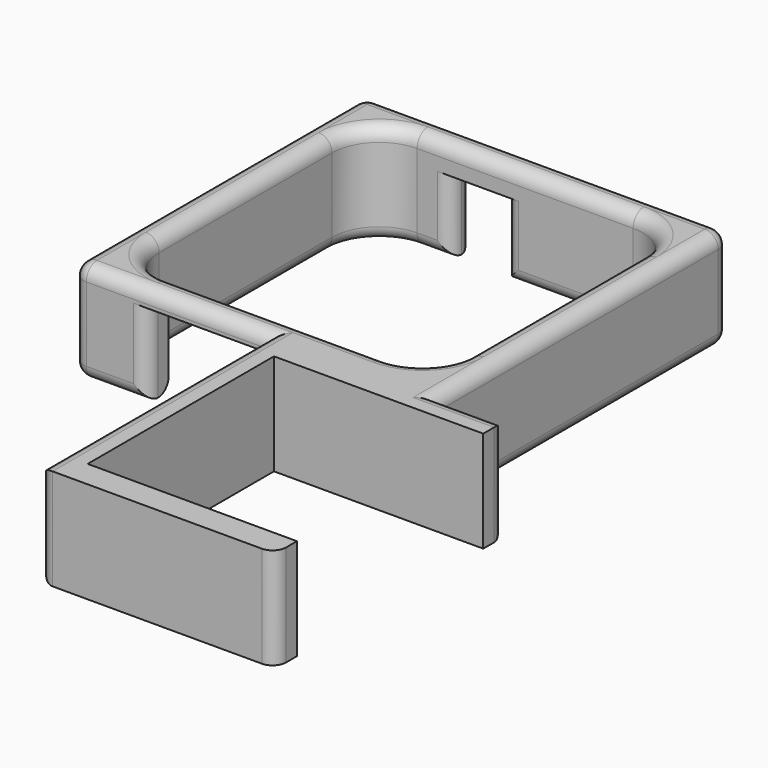
from build123d import *

# Parameters (mm, degrees)
F1_DEPTH = 7.5
F2_W     = 18
F2_H     = 4
F2_W_2   = 8
F3_DEPTH = 7.5
F4_DEPTH = 5
F5_DEPTH = 25
F6_DEPTH = 3.5
F7_DEPTH = 25
F8_R     = 7
F9_R     = 1.99999


# Not quite as in the source:
# - a fillet or chamfer is up to 0.001 mm smaller than in the source, because OpenCascade refuses the exact size


with BuildPart() as f1:
    # F0 (on Top) → F1 (new body, symmetric)
    with BuildSketch(Plane.XY):
        Polygon((29.4704200836, 10.5355388032), (29.4704200836, 14.5355388032), (-5.5295799164, 14.5355388032), (-5.5295799164, -27.9644611968), (29.4704200836, -27.9644611968), (29.4704200836, -23.9644611968), (27.4704200836, -23.9644611968), (-1.5295799164, -23.9644611968), (-1.5295799164, 10.5355388032), (27.4704200836, 10.5355388032), align=None)
    extrude(amount=F1_DEPTH, both=True)

    # F2 (on Top) → F3 (join, symmetric)
    with BuildSketch(Plane.XY):
        Polygon((-30.5295799164, 18.5355388032), (-30.5295799164, 64.5355388032), (-18.5295799164, 64.5355388032), (-18.5295799164, 68.5355388032), (-34.5295799164, 68.5355388032), (-34.5295799164, 14.5355388032), (-23.5295799164, 14.5355388032), (-23.5295799164, 18.5355388032), align=None)
        Polygon((-10.5295799164, 68.5355388032), (-10.5295799164, 64.5355388032), (15.4704200836, 64.5355388032), (15.4704200836, 18.5355388032), (-5.5295799164, 18.5355388032), (-5.5295799164, 14.5355388032), (19.4704200836, 14.5355388032), (19.4704200836, 68.5355388032), align=None)
        with Locations((-14.5295799164, 16.5355388032)):
            Rectangle(F2_W, F2_H)
        with Locations((-14.5295799164, 66.5355388032)):
            Rectangle(F2_W_2, F2_H)
    extrude(amount=F3_DEPTH, both=True)

    # F2 (on Top) → F4 (cut, symmetric)
    with BuildSketch(Plane.XY):
        with Locations((-14.5295799164, 16.5355388032)):
            Rectangle(F2_W, F2_H)
    extrude(amount=F4_DEPTH, both=True, mode=Mode.SUBTRACT)

    # F2 (on Top) → F5 (cut)
    with BuildSketch(Plane.XY):
        with Locations((-14.5295799164, 16.5355388032)):
            Rectangle(F2_W, F2_H)
    extrude(amount=-F5_DEPTH, mode=Mode.SUBTRACT)

    # F2 (on Top) → F6 (cut, symmetric)
    with BuildSketch(Plane.XY):
        with Locations((-14.5295799164, 66.5355388032)):
            Rectangle(F2_W_2, F2_H)
    extrude(amount=F6_DEPTH, both=True, mode=Mode.SUBTRACT)

    # F2 (on Top) → F7 (cut)
    with BuildSketch(Plane.XY):
        with Locations((-14.5295799164, 66.5355388032)):
            Rectangle(F2_W_2, F2_H)
    extrude(amount=-F7_DEPTH, mode=Mode.SUBTRACT)

    # F8
    f8_edges = [f1.edges().sort_by_distance(p)[0] for p in [
        (-30.52958, 64.535539, 0),
        (15.47042, 64.535539, 0),
        (-30.52958, 18.535539, 0),
        (15.47042, 18.535539, 0),
    ]]
    fillet(f8_edges, radius=F8_R)

    # F9 (radius 2 in the source; OpenCascade refuses exactly that, so slightly less here)
    f9_edges = [f1.edges().sort_by_distance(p)[0] for p in [
        (19.47042, 41.535539, 7.5),
        (19.47042, 41.535539, -7.5),
        (24.47042, 14.535539, 7.5),
        (24.47042, 14.535539, -7.5),
        (19.47042, 68.535539, 0),
        (4.47042, 68.535539, -7.5),
        (-7.52958, 68.535539, 7.5),
        (-14.52958, 68.535539, 3.5),
        (-18.52958, 68.535539, -2),
        (-10.52958, 68.535539, -2),
        (-10.52958, 64.535539, -2),
        (-18.52958, 64.535539, -2),
        (-34.52958, 68.535539, 0),
        (-26.52958, 68.535539, -7.5),
        (-30.52958, 41.535539, -7.5),
        (15.47042, 41.535539, -7.5),
        (-34.52958, 41.535539, -7.5),
        (-29.02958, 14.535539, -7.5),
        (-34.52958, 41.535539, 7.5),
        (-20.02958, 14.535539, 7.5),
        (-30.52958, 41.535539, 7.5),
        (-23.52958, 14.535539, -1.25),
        (-5.52958, 18.535539, -1.25),
        (-5.52958, -4.714461, -7.5),
        (-5.52958, -6.714461, 7.5),
        (29.47042, -27.964461, 0),
        (-5.52958, -27.964461, 0),
        (-34.52958, 14.535539, 0),
        (29.47042, 14.535539, 0),
        (-21.02958, 64.535539, -7.5),
        (-28.479327, 62.485286, -7.5),
        (-28.479327, 20.585791, -7.5),
        (-28.479327, 20.585791, 7.5),
        (-7.52958, 64.535539, 7.5),
        (-1.02958, 64.535539, -7.5),
        (-28.479327, 62.485286, 7.5),
        (-7.52958, 18.535539, 7.5),
        (13.420168, 20.585791, 7.5),
        (13.420168, 62.485286, 7.5),
        (15.47042, 41.535539, 7.5),
        (1.47042, 18.535539, -7.5),
        (13.420168, 62.485286, -7.5),
        (13.420168, 20.585791, -7.5),
    ]]
    fillet(f9_edges, radius=F9_R)


solid = f1.part
